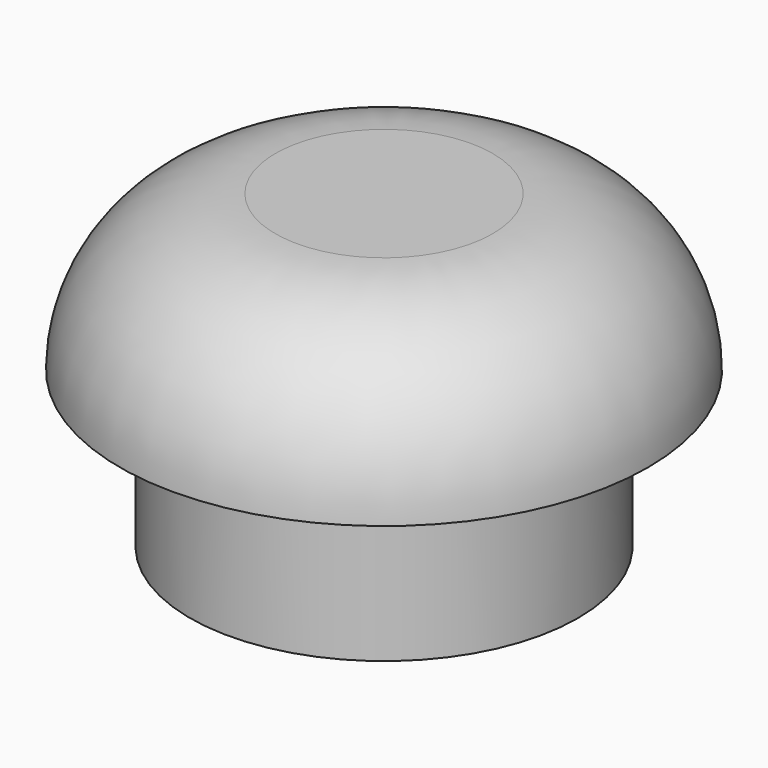
from build123d import *

# Parameters (mm, degrees)
F0_R     = 15.875
F1_DEPTH = 12.7
F2_R     = 21.59
F2_R_2   = 15.875
F3_DEPTH = 12.7
F4_R     = 12.69999


# Not quite as in the source:
# - a fillet or chamfer is up to 0.001 mm smaller than in the source, because OpenCascade refuses the exact size


with BuildPart() as f1:
    # F0 (on Top) → F1 (new body)
    with BuildSketch(Plane.XY):
        Circle(F0_R)
    extrude(amount=F1_DEPTH)

    # F2 (on face) → F3 (join)
    with BuildSketch(Plane.XY.offset(12.7)):
        Circle(F2_R)
        Circle(F2_R_2, mode=Mode.SUBTRACT)
        Circle(F2_R_2)
    extrude(amount=F3_DEPTH)

    # F4 (radius 12.7 in the source; OpenCascade refuses exactly that, so slightly less here)
    f4_edges = [f1.edges().sort_by_distance(p)[0] for p in [
        (-21.59, 0, 25.4),
    ]]
    fillet(f4_edges, radius=F4_R)


solid = f1.part
